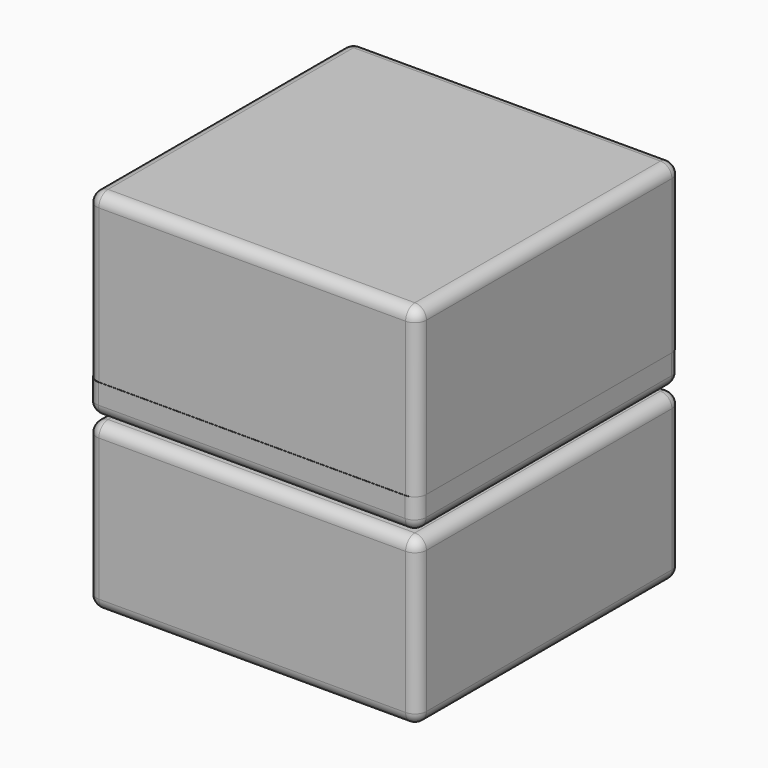
from build123d import *

# Parameters (mm, degrees)
F0_R          = 13.5
F0_R_2        = 12.5
F1_DEPTH      = 5
F3_R          = 12
F4_DEPTH      = 3.5
F5_R          = 12.5
F5_R_2        = 3.75
F6_DEPTH      = 0.5
F8_R          = 13.5
F9_DEPTH      = 0.5
F10_R         = 3.25
F11_DEPTH     = 2
F13_W         = 57
F13_H         = 57
F14_DEPTH     = 28.5
F15_R         = 2
F17_W         = 57
F17_H         = 57
F18_DEPTH     = 28.5
F19_W         = 57
F19_H         = 57
F19_R         = 13.5
F20_DEPTH     = 5.5
F21_T1_DEPTH  = 26.5
F21_T3_DEPTH  = 5.5
F21_T5_DEPTH  = 53
F21_T7_DEPTH  = 53
F21_S11_W     = 2.04
F21_S11_H     = 2.04
F21_T12_DEPTH = 2.04
F21_S17_W     = 2.04
F21_S17_H     = 2.04
F21_T18_DEPTH = 2.04
F21_S23_W     = 2.04
F21_S23_H     = 2.04
F21_T24_DEPTH = 2.04
F21_S29_W     = 2.04
F21_S29_H     = 2.04
F21_T30_DEPTH = 2.04
F22_T1_DEPTH  = 3.5
F22_T3_DEPTH  = 8.5
F22_T5_DEPTH  = 53
F22_T7_DEPTH  = 53
F22_S11_W     = 2.04
F22_S11_H     = 2.04
F22_T12_DEPTH = 2.04
F22_S17_W     = 2.04
F22_S17_H     = 2.04
F22_T18_DEPTH = 2.04
F22_S23_W     = 2.04
F22_S23_H     = 2.04
F22_T24_DEPTH = 2.04
F22_T28_ANGLE = 89.9999999955


# Not quite as in the source:
# - a fillet or chamfer that OpenCascade refuses, or shapes differently, is made with other operations: its cross-section is extruded or revolved along the edge and cut away or added


with BuildPart() as f1:
    # F0 (on Top) → F1 (new body)
    with BuildSketch(Plane.XY):
        Circle(F0_R)
        Circle(F0_R_2, mode=Mode.SUBTRACT)
    extrude(amount=F1_DEPTH)

    # F5 (on Top) → F6 (join)
    with BuildSketch(Plane.XY):
        Circle(F5_R)
        Circle(F5_R_2, mode=Mode.SUBTRACT)
    extrude(amount=F6_DEPTH)

    # F8 (on offset) → F9 (join)
    with BuildSketch(Plane.XY.offset(5)):
        Circle(F8_R)
    extrude(amount=F9_DEPTH)

    # F17 (on offset) → F18 (join)
    with BuildSketch(Plane.XY.offset(5.5)):
        Rectangle(F17_W, F17_H)
    extrude(amount=F18_DEPTH)

    # F19 (on offset) → F20 (join)
    with BuildSketch(Plane.XY.offset(5.5)):
        with Locations((-0.0443849862, -0.0324733704)):
            Rectangle(F19_W, F19_H)
        Circle(F19_R, mode=Mode.SUBTRACT)
    extrude(amount=-F20_DEPTH)

    # F21: fillet of radius 2 on 9 edges, made by hand

    # F21_s2 → F21_t1 (cut)
    with BuildSketch(Plane.XY.offset(5.5)):
        with BuildLine():
            ThreePointArc((26.5, 28.5), (27.9142135624, 27.9142135624), (28.5, 26.5))
            Line((28.5, 26.5), (28.54, 26.5))
            Line((28.54, 26.5), (28.54, 28.54))
            Line((28.54, 28.54), (26.5, 28.54))
            Line((26.5, 28.54), (26.5, 28.5))
        make_face()
        with BuildLine():
            ThreePointArc((28.5, -26.5), (27.9142135624, -27.9142135624), (26.5, -28.5))
            Line((26.5, -28.5), (26.5, -28.54))
            Line((26.5, -28.54), (28.54, -28.54))
            Line((28.54, -28.54), (28.54, -26.5))
            Line((28.54, -26.5), (28.5, -26.5))
        make_face()
        with BuildLine():
            ThreePointArc((-28.5, -26.5), (-27.9142135624, -27.9142135624), (-26.5, -28.5))
            Line((-26.5, -28.5), (-26.5, -28.54))
            Line((-26.5, -28.54), (-28.54, -28.54))
            Line((-28.54, -28.54), (-28.54, -26.5))
            Line((-28.54, -26.5), (-28.5, -26.5))
        make_face()
        with BuildLine():
            ThreePointArc((-26.5, 28.5), (-27.9142135624, 27.9142135624), (-28.5, 26.5))
            Line((-28.5, 26.5), (-28.54, 26.5))
            Line((-28.54, 26.5), (-28.54, 28.54))
            Line((-28.54, 28.54), (-26.5, 28.54))
            Line((-26.5, 28.54), (-26.5, 28.5))
        make_face()
    extrude(amount=F21_T1_DEPTH, mode=Mode.SUBTRACT)

    # F21_s4 → F21_t3 (cut)
    with BuildSketch(Plane.XY):
        with BuildLine():
            ThreePointArc((28.4556150138, 26.4675266296), (27.8698285762, 27.8817401919), (26.4556150138, 28.4675266296))
            Line((26.4556150138, 28.4675266296), (26.4556150138, 28.5075266296))
            Line((26.4556150138, 28.5075266296), (28.4956150138, 28.5075266296))
            Line((28.4956150138, 28.5075266296), (28.4956150138, 26.4675266296))
            Line((28.4956150138, 26.4675266296), (28.4556150138, 26.4675266296))
        make_face()
    extrude(amount=F21_T3_DEPTH, mode=Mode.SUBTRACT)

    # F21_s6 → F21_t5 (cut)
    with BuildSketch(Plane.YZ.offset(-26.5)):
        with BuildLine():
            ThreePointArc((28.5, 32), (27.9142135624, 33.4142135624), (26.5, 34))
            Line((26.5, 34), (26.5, 34.04))
            Line((26.5, 34.04), (28.54, 34.04))
            Line((28.54, 34.04), (28.54, 32))
            Line((28.54, 32), (28.5, 32))
        make_face()
        with BuildLine():
            ThreePointArc((-26.5, 34), (-27.9142135624, 33.4142135624), (-28.5, 32))
            Line((-28.5, 32), (-28.54, 32))
            Line((-28.54, 32), (-28.54, 34.04))
            Line((-28.54, 34.04), (-26.5, 34.04))
            Line((-26.5, 34.04), (-26.5, 34))
        make_face()
    extrude(amount=F21_T5_DEPTH, mode=Mode.SUBTRACT)

    # F21_s8 → F21_t7 (cut)
    with BuildSketch(Plane.XZ.offset(-26.5)):
        with BuildLine():
            ThreePointArc((-28.5, 32), (-27.9142135624, 33.4142135624), (-26.5, 34))
            Line((-26.5, 34), (-26.5, 34.04))
            Line((-26.5, 34.04), (-28.54, 34.04))
            Line((-28.54, 34.04), (-28.54, 32))
            Line((-28.54, 32), (-28.5, 32))
        make_face()
        with BuildLine():
            ThreePointArc((28.5, 32), (27.9142135624, 33.4142135624), (26.5, 34))
            Line((26.5, 34), (26.5, 34.04))
            Line((26.5, 34.04), (28.54, 34.04))
            Line((28.54, 34.04), (28.54, 32))
            Line((28.54, 32), (28.5, 32))
        make_face()
    extrude(amount=F21_T7_DEPTH, mode=Mode.SUBTRACT)


with BuildPart() as f4:
    # F3 (on offset) → F4 (new body)
    with BuildSketch(Plane.XY.offset(1)):
        Circle(F3_R)
    extrude(amount=F4_DEPTH)

    # F10 (on offset) → F11 (join)
    with BuildSketch(Plane.XY.offset(1)):
        Circle(F10_R)
    extrude(amount=-F11_DEPTH)

    # F13 (on offset) → F14 (join)
    with BuildSketch(Plane.XY.offset(-1)):
        Rectangle(F13_W, F13_H)
    extrude(amount=-F14_DEPTH)

    # F15
    f15_edges = [f4.edges().sort_by_distance(p)[0] for p in [
        (28.5, 0, -1),
        (-28.5, 0, -1),
        (0, -28.5, -1),
        (0, 28.5, -1),
        (-28.5, 28.5, -15.25),
        (28.5, 28.5, -15.25),
        (-28.5, -28.5, -15.25),
        (28.5, -28.5, -15.25),
        (-28.5, 0, -29.5),
        (0, -28.5, -29.5),
        (28.5, 0, -29.5),
        (0, 28.5, -29.5),
    ]]
    fillet(f15_edges, radius=F15_R)


with BuildPart() as f21_tool10:
    # F21_s11 → F21_t12 (new body)
    with BuildSketch(Plane.XZ.offset(-26.5)):
        with Locations((27.52, 33.02)):
            Rectangle(F21_S11_W, F21_S11_H)
    extrude(amount=-F21_T12_DEPTH)

    # F21_s13 → F21_t14 (revolve, cut)
    with BuildSketch(Plane(origin=(26.5, 26.5, 32), x_dir=(-0.7071067812, 0, -0.7071067812), z_dir=(0.7071067812, 0, -0.7071067812))):
        with BuildLine():
            ThreePointArc((0, -2), (2, 0), (0, 2))
            Line((0, 2), (0, -2))
        make_face()
    revolve(axis=Axis((26.5, 26.5, 32), (0, 1, 0)), mode=Mode.SUBTRACT)


with BuildPart() as f1_1:
    add(f1.part)

    # F21_t9: cut F21_tool10
    add(f21_tool10.part, mode=Mode.SUBTRACT)


with BuildPart() as f21_tool16:
    # F21_s17 → F21_t18 (new body)
    with BuildSketch(Plane.XZ.offset(-26.5)):
        with Locations((-27.52, 33.02)):
            Rectangle(F21_S17_W, F21_S17_H)
    extrude(amount=-F21_T18_DEPTH)

    # F21_s19 → F21_t20 (revolve, cut)
    with BuildSketch(Plane(origin=(-26.5, 26.5, 32), x_dir=(0.7071067812, 0, -0.7071067812), z_dir=(0.7071067812, 0, 0.7071067812))):
        with BuildLine():
            ThreePointArc((0, -2), (2, 0), (0, 2))
            Line((0, 2), (0, -2))
        make_face()
    revolve(axis=Axis((-26.5, 26.5, 32), (0, 1, 0)), mode=Mode.SUBTRACT)


with BuildPart() as f1_2:
    add(f1_1.part)

    # F21_t15: cut F21_tool16
    add(f21_tool16.part, mode=Mode.SUBTRACT)


with BuildPart() as f21_tool22:
    # F21_s23 → F21_t24 (new body)
    with BuildSketch(Plane.YZ.offset(-26.5)):
        with Locations((-27.52, 33.02)):
            Rectangle(F21_S23_W, F21_S23_H)
    extrude(amount=-F21_T24_DEPTH)

    # F21_s25 → F21_t26 (revolve, cut)
    with BuildSketch(Plane(origin=(-26.5, -26.5, 32), x_dir=(0, 0.7071067812, -0.7071067812), z_dir=(0, 0.7071067812, 0.7071067812))):
        with BuildLine():
            ThreePointArc((0, -2), (2, 0), (0, 2))
            Line((0, 2), (0, -2))
        make_face()
    revolve(axis=Axis((-26.5, -26.5, 32), (-1, 0, 0)), mode=Mode.SUBTRACT)


with BuildPart() as f1_3:
    add(f1_2.part)

    # F21_t21: cut F21_tool22
    add(f21_tool22.part, mode=Mode.SUBTRACT)


with BuildPart() as f21_tool28:
    # F21_s29 → F21_t30 (new body)
    with BuildSketch(Plane.YZ.offset(26.5)):
        with Locations((-27.52, 33.02)):
            Rectangle(F21_S29_W, F21_S29_H)
    extrude(amount=F21_T30_DEPTH)

    # F21_s31 → F21_t32 (revolve, cut)
    with BuildSketch(Plane(origin=(26.5, -26.5, 32), x_dir=(0, 0.7071067812, -0.7071067812), z_dir=(0, -0.7071067812, -0.7071067812))):
        with BuildLine():
            ThreePointArc((0, -2), (2, 0), (0, 2))
            Line((0, 2), (0, -2))
        make_face()
    revolve(axis=Axis((26.5, -26.5, 32), (1, 0, 0)), mode=Mode.SUBTRACT)


with BuildPart() as f1_4:
    add(f1_3.part)

    # F21_t27: cut F21_tool28
    add(f21_tool28.part, mode=Mode.SUBTRACT)

    # F22: fillet of radius 2 on 9 edges, made by hand

    # F22_s2 → F22_t1 (cut)
    with BuildSketch(Plane.XY.offset(2)):
        with BuildLine():
            ThreePointArc((28.4556150138, -26.5324733704), (27.8698285762, -27.9466869328), (26.4556150138, -28.5324733704))
            Line((26.4556150138, -28.5324733704), (28.4556150138, -28.5324733704))
            Line((28.4556150138, -28.5324733704), (28.4556150138, -26.5324733704))
        make_face()
        with BuildLine():
            ThreePointArc((-26.5443849862, 28.4675266296), (-27.9585985485, 27.8817401919), (-28.5443849862, 26.4675266296))
            Line((-28.5443849862, 26.4675266296), (-28.5443849862, 28.4675266296))
            Line((-28.5443849862, 28.4675266296), (-26.5443849862, 28.4675266296))
        make_face()
    extrude(amount=F22_T1_DEPTH, mode=Mode.SUBTRACT)

    # F22_s4 → F22_t3 (cut)
    with BuildSketch(Plane.XY.offset(2)):
        with BuildLine():
            ThreePointArc((-28.5443849862, -26.5324733704), (-27.9585985485, -27.9466869328), (-26.5443849862, -28.5324733704))
            Line((-26.5443849862, -28.5324733704), (-28.5443849862, -28.5324733704))
            Line((-28.5443849862, -28.5324733704), (-28.5443849862, -26.5324733704))
        make_face()
    extrude(amount=F22_T3_DEPTH, mode=Mode.SUBTRACT)

    # F22_s6 → F22_t5 (cut)
    with BuildSketch(Plane.YZ.offset(-26.5443849862)):
        with BuildLine():
            ThreePointArc((28.4675266296, 2), (27.8817401919, 0.5857864376), (26.4675266296, 0))
            Line((26.4675266296, 0), (28.4675266296, 0))
            Line((28.4675266296, 0), (28.4675266296, 2))
        make_face()
        with BuildLine():
            ThreePointArc((-26.5324733704, 0), (-27.9466869328, 0.5857864376), (-28.5324733704, 2))
            Line((-28.5324733704, 2), (-28.5324733704, 0))
            Line((-28.5324733704, 0), (-26.5324733704, 0))
        make_face()
    extrude(amount=F22_T5_DEPTH, mode=Mode.SUBTRACT)

    # F22_s8 → F22_t7 (cut)
    with BuildSketch(Plane.XZ.offset(-26.4675266296)):
        with BuildLine():
            ThreePointArc((28.4556150138, 2), (27.8698285762, 0.5857864376), (26.4556150138, 0))
            Line((26.4556150138, 0), (28.4556150138, 0))
            Line((28.4556150138, 0), (28.4556150138, 2))
        make_face()
        with BuildLine():
            ThreePointArc((-28.5443849862, 2), (-27.9585985485, 0.5857864376), (-26.5443849862, 0))
            Line((-26.5443849862, 0), (-28.5443849862, 0))
            Line((-28.5443849862, 0), (-28.5443849862, 2))
        make_face()
    extrude(amount=F22_T7_DEPTH, mode=Mode.SUBTRACT)


with BuildPart() as f22_tool10:
    # F22_s11 → F22_t12 (new body)
    with BuildSketch(Plane.XY.offset(2)):
        with Locations((27.4756150138, -27.5524733704)):
            Rectangle(F22_S11_W, F22_S11_H)
    extrude(amount=-F22_T12_DEPTH)

    # F22_s13 → F22_t14 (revolve, cut)
    with BuildSketch(Plane(origin=(26.4556150138, -26.5324733704, 2), x_dir=(-0.7071067812, 0.7071067812, 0), z_dir=(-0.7071067812, -0.7071067812, 0))):
        with BuildLine():
            ThreePointArc((0, -2), (2, 0), (0, 2))
            Line((0, 2), (0, -2))
        make_face()
    revolve(axis=Axis((26.4556150138, -26.5324733704, 2), (0, 0, -1)), mode=Mode.SUBTRACT)


with BuildPart() as f1_5:
    add(f1_4.part)

    # F22_t9: cut F22_tool10
    add(f22_tool10.part, mode=Mode.SUBTRACT)


with BuildPart() as f22_tool16:
    # F22_s17 → F22_t18 (new body)
    with BuildSketch(Plane.YZ.offset(-26.5443849862)):
        with Locations((-27.5524733704, 0.98)):
            Rectangle(F22_S17_W, F22_S17_H)
    extrude(amount=-F22_T18_DEPTH)

    # F22_s19 → F22_t20 (revolve, cut)
    with BuildSketch(Plane(origin=(-26.5443849862, -26.5324733704, 2), x_dir=(0, 0.7071067812, 0.7071067812), z_dir=(0, -0.7071067812, 0.7071067812))):
        with BuildLine():
            ThreePointArc((0, -2), (2, 0), (0, 2))
            Line((0, 2), (0, -2))
        make_face()
    revolve(axis=Axis((-26.5443849862, -26.5324733704, 2), (-1, 0, 0)), mode=Mode.SUBTRACT)


with BuildPart() as f1_6:
    add(f1_5.part)

    # F22_t15: cut F22_tool16
    add(f22_tool16.part, mode=Mode.SUBTRACT)


with BuildPart() as f22_tool22:
    # F22_s23 → F22_t24 (new body)
    with BuildSketch(Plane.XZ.offset(-26.4675266296)):
        with Locations((-27.5643849862, 0.98)):
            Rectangle(F22_S23_W, F22_S23_H)
    extrude(amount=-F22_T24_DEPTH)

    # F22_s25 → F22_t26 (revolve, cut)
    with BuildSketch(Plane(origin=(-26.5443849862, 26.4675266296, 2), x_dir=(0.7071067812, 0, 0.7071067812), z_dir=(-0.7071067812, 0, 0.7071067812))):
        with BuildLine():
            ThreePointArc((0, -2), (2, 0), (0, 2))
            Line((0, 2), (0, -2))
        make_face()
    revolve(axis=Axis((-26.5443849862, 26.4675266296, 2), (0, 1, 0)), mode=Mode.SUBTRACT)


with BuildPart() as f1_7:
    add(f1_6.part)

    # F22_t21: cut F22_tool22
    add(f22_tool22.part, mode=Mode.SUBTRACT)

    # F22_s27 → F22_t28 (revolve, cut)
    with BuildSketch(Plane.XZ.offset(-26.4675266295)):
        with BuildLine():
            ThreePointArc((28.4556150138, 2), (27.8698285762, 0.5857864376), (26.4556150138, 0))
            Line((26.4556150138, 0), (28.4556150138, 0))
            Line((28.4556150138, 0), (28.4556150138, 2))
        make_face()
    revolve(axis=Axis((26.4556150137, 26.4675266295, 0), (0, 0, 1)), revolution_arc=F22_T28_ANGLE, mode=Mode.SUBTRACT)

    # F22_s29 → F22_t30 (revolve, cut)
    with BuildSketch(Plane.XZ):
        with BuildLine():
            ThreePointArc((5.0728756555, 0), (4.3657688743, 0.1291713066), (3.75, 0.5))
            Line((3.75, 0.5), (3.75, 0))
            Line((3.75, 0), (5.0728756555, 0))
        make_face()
    revolve(axis=Axis((0, 0, 0), (0, 0, 1)), mode=Mode.SUBTRACT)


solid = Compound([f4.part, f1_7.part])
